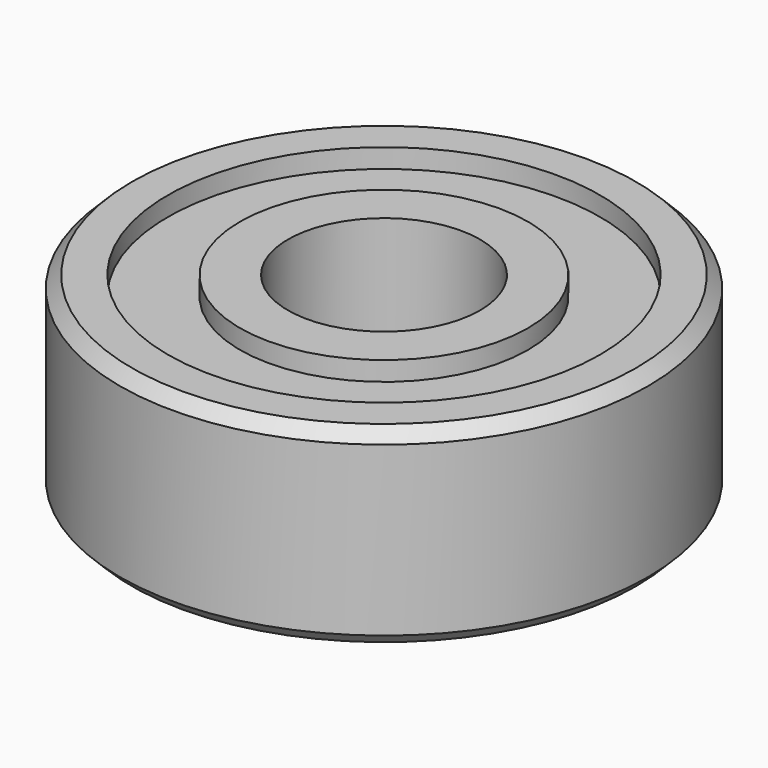
from build123d import *

# Parameters (mm, degrees)
F0_R     = 11
F0_R_2   = 4
F1_DEPTH = 4
F2_R     = 9
F2_R_2   = 6
F3_DEPTH = 0.8
F4_SIZE  = 0.5


# Not quite as in the source:
# - a pattern or mirror of a feature is missing from the dataset's text; its kind, count and spacing are read off the source's solid


with BuildPart() as f1:
    # F0 (on Top) → F1 (new body, symmetric)
    with BuildSketch(Plane.XY):
        Circle(F0_R)
        Circle(F0_R_2, mode=Mode.SUBTRACT)
    extrude(amount=F1_DEPTH, both=True)

    # F2 (on face) → F3 (cut)
    with BuildSketch(Plane.XY.offset(4)):
        Circle(F2_R)
        Circle(F2_R_2, mode=Mode.SUBTRACT)
    f3 = extrude(amount=-F3_DEPTH, mode=Mode.SUBTRACT)

    # F3_copies: F3 across plane
    add(f3.mirror(Plane(origin=(0, 0, 0), x_dir=(-1, 0, 0), z_dir=(0, 0, -1))), mode=Mode.SUBTRACT)

    # F4
    f4_edges = [f1.edges().sort_by_distance(p)[0] for p in [
        (-11, 0, 4),
        (-11, 0, -4),
    ]]
    chamfer(f4_edges, length=F4_SIZE)


solid = f1.part
